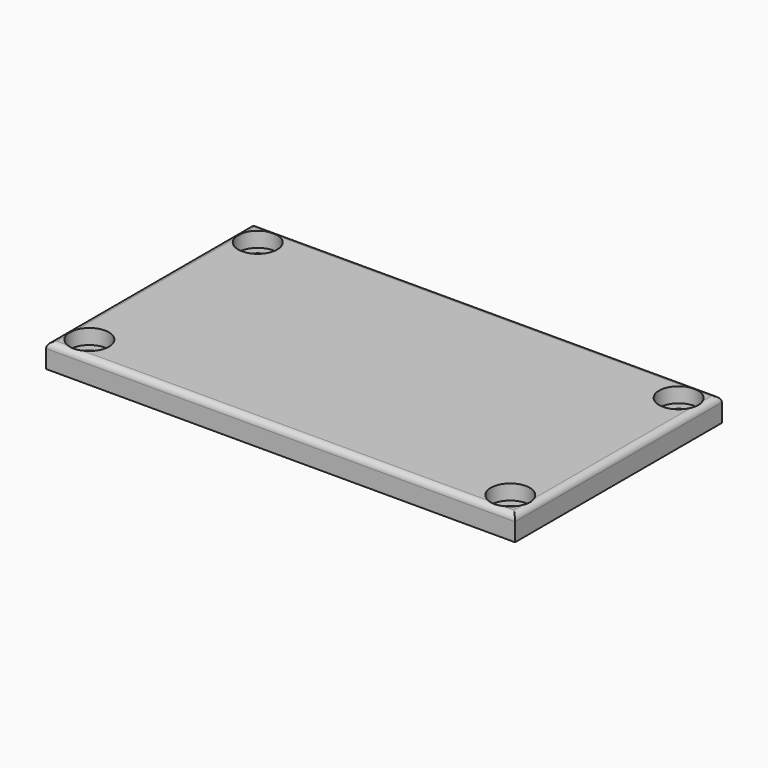
from build123d import *

# Parameters (mm, degrees)
F0_W        = 78
F0_H        = 43
F1_DEPTH    = 4
F2_R        = 1.75
F3_DEPTH    = 4.001
F4_R        = 3.25
F5_DEPTH    = 2.5
F6_T1_DEPTH = 48
F6_T3_DEPTH = 83


# Not quite as in the source:
# - a fillet or chamfer that OpenCascade refuses, or shapes differently, is made with other operations: its cross-section is extruded or revolved along the edge and cut away or added


with BuildPart() as f1:
    # F0 (on Top) → F1 (new body)
    with BuildSketch(Plane.XY):
        with Locations((34.9585738778, -17.5538536012)):
            Rectangle(F0_W, F0_H)
    extrude(amount=F1_DEPTH)

    # F2 (on face) → F3 (cut, through all)
    with BuildSketch(Plane.XY.offset(4)):
        with Locations((-0.0414261222, -0.0538536012)):
            Circle(F2_R)
        with Locations((69.9585738778, -0.0538536012)):
            Circle(F2_R)
        with Locations((69.9585738778, -35.0538536012)):
            Circle(F2_R)
        with Locations((-0.0414261222, -35.0538536012)):
            Circle(F2_R)
    extrude(amount=-F3_DEPTH, mode=Mode.SUBTRACT)

    # F4 (on face) → F5 (cut)
    with BuildSketch(Plane.XY.offset(4)):
        with Locations((-0.0414261222, -0.0538536012)):
            Circle(F4_R)
        with Locations((69.9585738778, -0.0538536012)):
            Circle(F4_R)
        with Locations((69.9585738778, -35.0538536012)):
            Circle(F4_R)
        with Locations((-0.0414261222, -35.0538536012)):
            Circle(F4_R)
    extrude(amount=-F5_DEPTH, mode=Mode.SUBTRACT)

    # F6: fillet of radius 1 on 4 edges, made by hand

    # F6_s2 → F6_t1 (cut)
    with BuildSketch(Plane.XZ.offset(-6.4461463988)):
        with BuildLine():
            ThreePointArc((-4.0414261222, 3), (-3.7485329034, 3.7071067812), (-3.0414261222, 4))
            Line((-3.0414261222, 4), (-4.0414261222, 4))
            Line((-4.0414261222, 4), (-4.0414261222, 3))
        make_face()
        with BuildLine():
            ThreePointArc((73.9585738778, 3), (73.665680659, 3.7071067812), (72.9585738778, 4))
            Line((72.9585738778, 4), (73.9585738778, 4))
            Line((73.9585738778, 4), (73.9585738778, 3))
        make_face()
    extrude(amount=F6_T1_DEPTH, mode=Mode.SUBTRACT)

    # F6_s4 → F6_t3 (cut)
    with BuildSketch(Plane.YZ.offset(-6.5414261222)):
        with BuildLine():
            ThreePointArc((-39.0538536012, 3), (-38.7609603824, 3.7071067812), (-38.0538536012, 4))
            Line((-38.0538536012, 4), (-39.0538536012, 4))
            Line((-39.0538536012, 4), (-39.0538536012, 3))
        make_face()
        with BuildLine():
            ThreePointArc((2.9461463988, 4), (3.65325318, 3.7071067812), (3.9461463988, 3))
            Line((3.9461463988, 3), (3.9461463988, 4))
            Line((3.9461463988, 4), (2.9461463988, 4))
        make_face()
    extrude(amount=F6_T3_DEPTH, mode=Mode.SUBTRACT)


solid = f1.part
